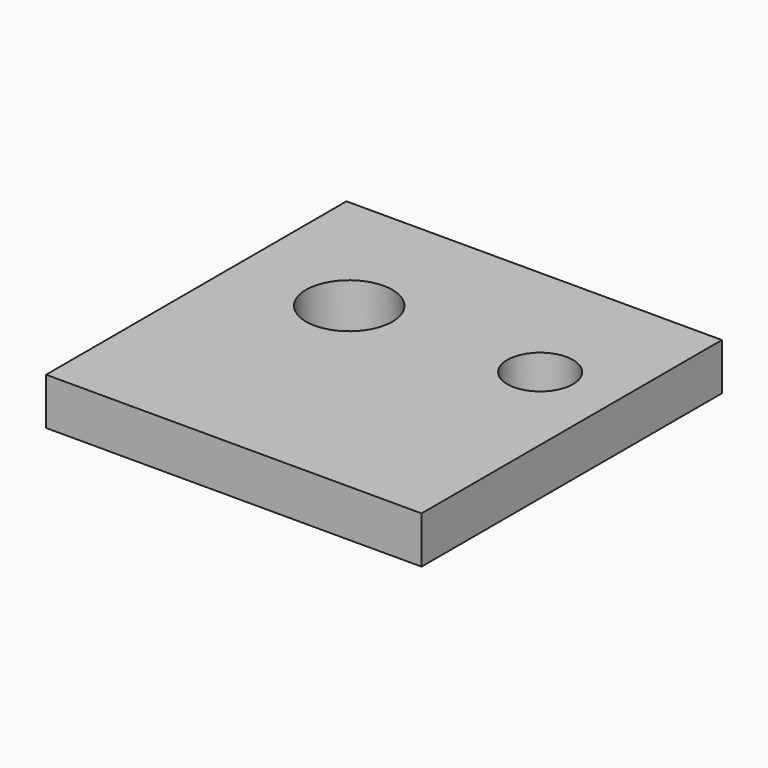
from build123d import *

# Parameters (mm, degrees)
F0_W     = 25.4
F0_H     = 25.4
F0_R     = 2.921
F0_R_2   = 2.2225
F1_DEPTH = 3.175


# Not quite as in the source:
# - a feature names something its author has since deleted; it is built from what else it names


with BuildPart() as f1:
    # F0 (on Top) → F1 (new body)
    with BuildSketch(Plane.XY):
        with Locations((-4.1276658885, 3.1854207028)):
            Rectangle(F0_W, F0_H)
        with Locations((-9.2504761174, 6.6469578254)):
            Circle(F0_R, mode=Mode.SUBTRACT)
        with Locations((3.3648989856, 7.0253587247)):
            Circle(F0_R_2, mode=Mode.SUBTRACT)
    extrude(amount=-F1_DEPTH)


solid = f1.part
